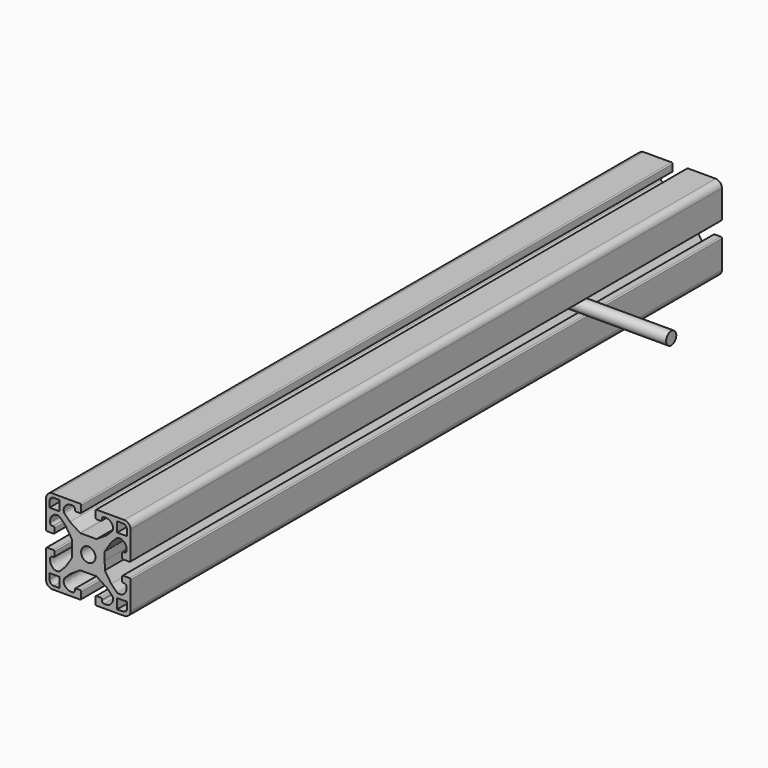
from build123d import *

# Parameters (mm, degrees)
F0_R     = 3.4
F1_DEPTH = 350
F2_R     = 3
F3_DEPTH = 60


with BuildPart() as f1:
    # F0 (on Front) → F1 (new body)
    with BuildSketch(Plane.XZ):
        with BuildLine():
            ThreePointArc((-18.3550221846, 16.3550221846), (-17.7692357469, 17.7692357469), (-16.3550221846, 18.3550221846))
            Line((-16.3550221846, 18.3550221846), (-14.0237337309, 18.3550221846))
            add(Edge.make_bspline(
                [(-14.0237337309, 18.3550221845), (-14.2706563501, 18.8700433502), (-14.531764339, 19.4199819881), (-14.8048075585, 20)],
                knots=[0.5315869177, 0.5315869177, 0.5315869177, 0.5315869177, 0.5531016129, 0.5531016129, 0.5531016129, 0.5531016129], degree=3))
            Line((-14.8048075585, 20), (-17, 20))
            ThreePointArc((-17, 20), (-19.1213203436, 19.1213203436), (-20, 17))
            Line((-20, 17), (-20, 14.8048075585))
            add(Edge.make_bspline(
                [(-18.3550221845, 14.0237337309), (-18.8700433502, 14.2706563501), (-19.4199819881, 14.531764339), (-20, 14.8048075585)],
                knots=[0.5315869177, 0.5315869177, 0.5315869177, 0.5315869177, 0.5531016129, 0.5531016129, 0.5531016129, 0.5531016129], degree=3))
            Line((-18.3550221846, 14.0237337309), (-18.3550221846, 16.3550221846))
        make_face()
        with BuildLine():
            add(Edge.make_bspline(
                [(-14.0237337309, 18.3550221845), (-14.2706563501, 18.8700433502), (-14.531764339, 19.4199819881), (-14.8048075585, 20)],
                knots=[0.5315869177, 0.5315869177, 0.5315869177, 0.5315869177, 0.5531016129, 0.5531016129, 0.5531016129, 0.5531016129], degree=3))
            Line((-14.0237337309, 18.3550221846), (-13.6494976468, 18.3550221846))
            Line((-13.6494976468, 18.3550221846), (-13.6494976468, 17.5788207647))
            add(Edge.make_bspline(
                [(-11.594085993, 14.1061210716), (-11.5738798381, 13.895961995), (-11.5790441073, 13.4753849368), (-12.6022550623, 15.4198368213), (-13.6494976468, 17.5788207647)],
                knots=[0.3845285295, 0.3845285295, 0.3845285295, 0.3845285295, 0.4230558589, 0.5203726283, 0.5203726283, 0.5203726283, 0.5203726283], degree=3))
            add(Edge.make_bspline(
                [(-7.3380557529, 18.077673873), (-7.938915425, 18.114965287), (-9.2671967698, 18.1126101908), (-10.8204009228, 17.1496223508), (-11.7986304949, 15.6154448581), (-11.6169304386, 14.3437203378), (-11.594085993, 14.1061210716)],
                knots=[0.041617921, 0.041617921, 0.041617921, 0.041617921, 0.1226487952, 0.2279423965, 0.3409707382, 0.3845285295, 0.3845285295, 0.3845285295, 0.3845285295], degree=3))
            ThreePointArc((-7.3380557529, 18.077673873), (-6.6713216598, 17.7644503609), (-6.4, 17.0795942618))
            Line((-6.4, 17.0795942618), (-6.4, 16.5))
            ThreePointArc((-6.4, 16.5), (-6.2535533906, 16.1464466094), (-5.9, 16))
            Line((-5.9, 16), (-3.9, 16))
            ThreePointArc((-3.9, 16), (-3.5464466094, 16.1464466094), (-3.4, 16.5))
            Line((-3.4, 16.5), (-3.4, 19.5))
            ThreePointArc((-3.4, 19.5), (-3.5464466094, 19.8535533906), (-3.9, 20))
            Line((-3.9, 20), (-14.8048075585, 20))
        make_face()
        with BuildLine():
            add(Edge.make_bspline(
                [(-11.594085993, 14.1061210716), (-11.5738798381, 13.895961995), (-11.5790441073, 13.4753849368), (-12.6022550623, 15.4198368213), (-13.6494976468, 17.5788207647)],
                knots=[0.3845285295, 0.3845285295, 0.3845285295, 0.3845285295, 0.4230558589, 0.5203726283, 0.5203726283, 0.5203726283, 0.5203726283], degree=3))
            Line((-13.6494976468, 17.5788207647), (-13.6494976468, 13.6494976468))
            Line((-13.6494976468, 13.6494976468), (-17.5788207647, 13.6494976468))
            add(Edge.make_bspline(
                [(-14.1061210716, 11.594085993), (-13.895961995, 11.5738798381), (-13.4753849368, 11.5790441073), (-15.4198368213, 12.6022550623), (-17.5788207647, 13.6494976468)],
                knots=[0.3845285295, 0.3845285295, 0.3845285295, 0.3845285295, 0.4230558589, 0.5203726283, 0.5203726283, 0.5203726283, 0.5203726283], degree=3))
            ThreePointArc((-14.1061210716, 11.594085993), (-13.7753216108, 11.5031614821), (-13.4947198987, 11.3057830914))
            Line((-13.4947198987, 11.3057830914), (-10.8786681667, 8.6897313595))
            Line((-10.8786681667, 8.6897313595), (-7.8307420977, 3.9992546314))
            ThreePointArc((-7.8307420977, 3.9992546314), (-7.7706103093, 3.8688917636), (-7.75, 3.7268159936))
            Line((-7.75, 3.7268159936), (-7.75, -3.7268159936))
            ThreePointArc((-7.75, -3.7268159936), (-7.7706103093, -3.8688917636), (-7.8307420977, -3.9992546314))
            Line((-7.8307420977, -3.9992546314), (-10.8786681667, -8.6897313595))
            Line((-10.8786681667, -8.6897313595), (-13.4947198987, -11.3057830914))
            ThreePointArc((-13.4947198987, -11.3057830914), (-13.7753216108, -11.5031614821), (-14.1061210716, -11.594085993))
            add(Edge.make_bspline(
                [(-14.1061210716, -11.594085993), (-13.895961995, -11.5738798381), (-13.4753849368, -11.5790441073), (-15.4198368213, -12.6022550623), (-17.5788207647, -13.6494976468)],
                knots=[0.3845285295, 0.3845285295, 0.3845285295, 0.3845285295, 0.4230558589, 0.5203726283, 0.5203726283, 0.5203726283, 0.5203726283], degree=3))
            Line((-17.5788207647, -13.6494976468), (-13.6494976468, -13.6494976468))
            Line((-13.6494976468, -13.6494976468), (-13.6494976468, -17.5788207647))
            add(Edge.make_bspline(
                [(-11.594085993, -14.1061210716), (-11.5738798381, -13.895961995), (-11.5790441073, -13.4753849368), (-12.6022550623, -15.4198368213), (-13.6494976468, -17.5788207647)],
                knots=[0.3845285295, 0.3845285295, 0.3845285295, 0.3845285295, 0.4230558589, 0.5203726283, 0.5203726283, 0.5203726283, 0.5203726283], degree=3))
            ThreePointArc((-11.594085993, -14.1061210716), (-11.5031614821, -13.7753216108), (-11.3057830914, -13.4947198987))
            Line((-11.3057830914, -13.4947198987), (-8.6897313595, -10.8786681667))
            Line((-8.6897313595, -10.8786681667), (-3.9992546314, -7.8307420977))
            ThreePointArc((-3.9992546314, -7.8307420977), (-3.8688917636, -7.7706103093), (-3.7268159936, -7.75))
            Line((-3.7268159936, -7.75), (0, -7.75))
            Line((0, -7.75), (3.7268159936, -7.75))
            ThreePointArc((3.7268159936, -7.75), (3.8688917636, -7.7706103093), (3.9992546314, -7.8307420977))
            Line((3.9992546314, -7.8307420977), (8.6897313595, -10.8786681667))
            Line((8.6897313595, -10.8786681667), (11.3057830914, -13.4947198987))
            ThreePointArc((11.3057830914, -13.4947198987), (11.5031614821, -13.7753216108), (11.594085993, -14.1061210716))
            add(Edge.make_bspline(
                [(11.594085993, -14.1061210716), (11.5738798381, -13.895961995), (11.5790441073, -13.4753849368), (12.6022550623, -15.4198368213), (13.6494976468, -17.5788207647)],
                knots=[0.3845285295, 0.3845285295, 0.3845285295, 0.3845285295, 0.4230558589, 0.5203726283, 0.5203726283, 0.5203726283, 0.5203726283], degree=3))
            Line((13.6494976468, -17.5788207647), (13.6494976468, -13.6494976468))
            Line((13.6494976468, -13.6494976468), (17.5788207647, -13.6494976468))
            add(Edge.make_bspline(
                [(14.1061210716, -11.594085993), (13.895961995, -11.5738798381), (13.4753849368, -11.5790441073), (15.4198368213, -12.6022550623), (17.5788207647, -13.6494976468)],
                knots=[0.3845285295, 0.3845285295, 0.3845285295, 0.3845285295, 0.4230558589, 0.5203726283, 0.5203726283, 0.5203726283, 0.5203726283], degree=3))
            ThreePointArc((14.1061210716, -11.594085993), (13.7753216108, -11.5031614821), (13.4947198987, -11.3057830914))
            Line((13.4947198987, -11.3057830914), (10.8786681667, -8.6897313595))
            Line((10.8786681667, -8.6897313595), (7.8307420977, -3.9992546314))
            Line((7.8307420977, -3.9992546314), (7.75, 0))
            Line((7.75, 0), (7.75, 3.7268159936))
            ThreePointArc((7.75, 3.7268159936), (7.7706103093, 3.8688917636), (7.8307420977, 3.9992546314))
            Line((7.8307420977, 3.9992546314), (10.8786681667, 8.6897313595))
            Line((10.8786681667, 8.6897313595), (13.4947198987, 11.3057830914))
            ThreePointArc((13.4947198987, 11.3057830914), (13.7753216108, 11.5031614821), (14.1061210716, 11.594085993))
            add(Edge.make_bspline(
                [(14.1061210716, 11.594085993), (13.895961995, 11.5738798381), (13.4753849368, 11.5790441073), (15.4198368213, 12.6022550623), (17.5788207647, 13.6494976468)],
                knots=[0.3845285295, 0.3845285295, 0.3845285295, 0.3845285295, 0.4230558589, 0.5203726283, 0.5203726283, 0.5203726283, 0.5203726283], degree=3))
            Line((17.5788207647, 13.6494976468), (13.6494976468, 13.6494976468))
            Line((13.6494976468, 13.6494976468), (13.6494976468, 17.5788207647))
            add(Edge.make_bspline(
                [(11.594085993, 14.1061210716), (11.5738798381, 13.895961995), (11.5790441073, 13.4753849368), (12.6022550623, 15.4198368213), (13.6494976468, 17.5788207647)],
                knots=[0.3845285295, 0.3845285295, 0.3845285295, 0.3845285295, 0.4230558589, 0.5203726283, 0.5203726283, 0.5203726283, 0.5203726283], degree=3))
            ThreePointArc((11.594085993, 14.1061210716), (11.5031614821, 13.7753216108), (11.3057830914, 13.4947198987))
            Line((11.3057830914, 13.4947198987), (8.6897313595, 10.8786681667))
            Line((8.6897313595, 10.8786681667), (3.9992546314, 7.8307420977))
            ThreePointArc((3.9992546314, 7.8307420977), (3.8688917636, 7.7706103093), (3.7268159936, 7.75))
            Line((3.7268159936, 7.75), (0, 7.75))
            Line((0, 7.75), (-3.7268159936, 7.75))
            ThreePointArc((-3.7268159936, 7.75), (-3.8688917636, 7.7706103093), (-3.9992546314, 7.8307420977))
            Line((-3.9992546314, 7.8307420977), (-8.6897313595, 10.8786681667))
            Line((-8.6897313595, 10.8786681667), (-11.3057830914, 13.4947198987))
            ThreePointArc((-11.3057830914, 13.4947198987), (-11.5031614821, 13.7753216108), (-11.594085993, 14.1061210716))
        make_face()
        Circle(F0_R, mode=Mode.SUBTRACT)
        with BuildLine():
            Line((-18.3550221846, 13.6494976468), (-18.3550221846, 14.0237337309))
            add(Edge.make_bspline(
                [(-18.3550221845, 14.0237337309), (-18.8700433502, 14.2706563501), (-19.4199819881, 14.531764339), (-20, 14.8048075585)],
                knots=[0.5315869177, 0.5315869177, 0.5315869177, 0.5315869177, 0.5531016129, 0.5531016129, 0.5531016129, 0.5531016129], degree=3))
            Line((-20, 14.8048075585), (-20, 3.9))
            ThreePointArc((-20, 3.9), (-19.8535533906, 3.5464466094), (-19.5, 3.4))
            Line((-19.5, 3.4), (-16.5, 3.4))
            ThreePointArc((-16.5, 3.4), (-16.1464466094, 3.5464466094), (-16, 3.9))
            Line((-16, 3.9), (-16, 5.9))
            ThreePointArc((-16, 5.9), (-16.1464466094, 6.2535533906), (-16.5, 6.4))
            Line((-16.5, 6.4), (-17.0795942618, 6.4))
            ThreePointArc((-17.0795942618, 6.4), (-17.7644503609, 6.6713216598), (-18.077673873, 7.3380557529))
            add(Edge.make_bspline(
                [(-18.077673873, 7.3380557529), (-18.114965287, 7.938915425), (-18.1126101908, 9.2671967698), (-17.1496223508, 10.8204009228), (-15.6154448581, 11.7986304949), (-14.3437203378, 11.6169304386), (-14.1061210716, 11.594085993)],
                knots=[0.041617921, 0.041617921, 0.041617921, 0.041617921, 0.1226487952, 0.2279423965, 0.3409707382, 0.3845285295, 0.3845285295, 0.3845285295, 0.3845285295], degree=3))
            add(Edge.make_bspline(
                [(-14.1061210716, 11.594085993), (-13.895961995, 11.5738798381), (-13.4753849368, 11.5790441073), (-15.4198368213, 12.6022550623), (-17.5788207647, 13.6494976468)],
                knots=[0.3845285295, 0.3845285295, 0.3845285295, 0.3845285295, 0.4230558589, 0.5203726283, 0.5203726283, 0.5203726283, 0.5203726283], degree=3))
            Line((-17.5788207647, 13.6494976468), (-18.3550221846, 13.6494976468))
        make_face()
        with BuildLine():
            add(Edge.make_bspline(
                [(7.3380557529, 18.077673873), (7.938915425, 18.114965287), (9.2671967698, 18.1126101908), (10.8204009228, 17.1496223508), (11.7986304949, 15.6154448581), (11.6169304386, 14.3437203378), (11.594085993, 14.1061210716)],
                knots=[0.041617921, 0.041617921, 0.041617921, 0.041617921, 0.1226487952, 0.2279423965, 0.3409707382, 0.3845285295, 0.3845285295, 0.3845285295, 0.3845285295], degree=3))
            add(Edge.make_bspline(
                [(11.594085993, 14.1061210716), (11.5738798381, 13.895961995), (11.5790441073, 13.4753849368), (12.6022550623, 15.4198368213), (13.6494976468, 17.5788207647)],
                knots=[0.3845285295, 0.3845285295, 0.3845285295, 0.3845285295, 0.4230558589, 0.5203726283, 0.5203726283, 0.5203726283, 0.5203726283], degree=3))
            Line((13.6494976468, 17.5788207647), (13.6494976468, 18.3550221846))
            Line((13.6494976468, 18.3550221846), (14.0237337309, 18.3550221846))
            add(Edge.make_bspline(
                [(14.0237337309, 18.3550221845), (14.2706563501, 18.8700433502), (14.531764339, 19.4199819881), (14.8048075585, 20)],
                knots=[0.5315869177, 0.5315869177, 0.5315869177, 0.5315869177, 0.5531016129, 0.5531016129, 0.5531016129, 0.5531016129], degree=3))
            Line((14.8048075585, 20), (3.9, 20))
            ThreePointArc((3.9, 20), (3.5464466094, 19.8535533906), (3.4, 19.5))
            Line((3.4, 19.5), (3.4, 16.5))
            ThreePointArc((3.4, 16.5), (3.5464466094, 16.1464466094), (3.9, 16))
            Line((3.9, 16), (5.9, 16))
            ThreePointArc((5.9, 16), (6.2535533906, 16.1464466094), (6.4, 16.5))
            Line((6.4, 16.5), (6.4, 17.0795942618))
            ThreePointArc((6.4, 17.0795942618), (6.6713216598, 17.7644503609), (7.3380557529, 18.077673873))
        make_face()
        with BuildLine():
            add(Edge.make_bspline(
                [(-14.1061210716, -11.594085993), (-13.895961995, -11.5738798381), (-13.4753849368, -11.5790441073), (-15.4198368213, -12.6022550623), (-17.5788207647, -13.6494976468)],
                knots=[0.3845285295, 0.3845285295, 0.3845285295, 0.3845285295, 0.4230558589, 0.5203726283, 0.5203726283, 0.5203726283, 0.5203726283], degree=3))
            add(Edge.make_bspline(
                [(-18.077673873, -7.3380557529), (-18.114965287, -7.938915425), (-18.1126101908, -9.2671967698), (-17.1496223508, -10.8204009228), (-15.6154448581, -11.7986304949), (-14.3437203378, -11.6169304386), (-14.1061210716, -11.594085993)],
                knots=[0.041617921, 0.041617921, 0.041617921, 0.041617921, 0.1226487952, 0.2279423965, 0.3409707382, 0.3845285295, 0.3845285295, 0.3845285295, 0.3845285295], degree=3))
            ThreePointArc((-18.077673873, -7.3380557529), (-17.7644503609, -6.6713216598), (-17.0795942618, -6.4))
            Line((-17.0795942618, -6.4), (-16.5, -6.4))
            ThreePointArc((-16.5, -6.4), (-16.1464466094, -6.2535533906), (-16, -5.9))
            Line((-16, -5.9), (-16, -3.9))
            ThreePointArc((-16, -3.9), (-16.1464466094, -3.5464466094), (-16.5, -3.4))
            Line((-16.5, -3.4), (-19.5, -3.4))
            ThreePointArc((-19.5, -3.4), (-19.8535533906, -3.5464466094), (-20, -3.9))
            Line((-20, -3.9), (-20, -14.8048075585))
            add(Edge.make_bspline(
                [(-18.3550221845, -14.0237337309), (-18.8700433502, -14.2706563501), (-19.4199819881, -14.531764339), (-20, -14.8048075585)],
                knots=[0.5315869177, 0.5315869177, 0.5315869177, 0.5315869177, 0.5531016129, 0.5531016129, 0.5531016129, 0.5531016129], degree=3))
            Line((-18.3550221846, -14.0237337309), (-18.3550221846, -13.6494976468))
            Line((-18.3550221846, -13.6494976468), (-17.5788207647, -13.6494976468))
        make_face()
        with BuildLine():
            add(Edge.make_bspline(
                [(14.0237337309, 18.3550221845), (14.2706563501, 18.8700433502), (14.531764339, 19.4199819881), (14.8048075585, 20)],
                knots=[0.5315869177, 0.5315869177, 0.5315869177, 0.5315869177, 0.5531016129, 0.5531016129, 0.5531016129, 0.5531016129], degree=3))
            Line((14.0237337309, 18.3550221846), (16.3550221846, 18.3550221846))
            ThreePointArc((16.3550221846, 18.3550221846), (17.7692357469, 17.7692357469), (18.3550221846, 16.3550221846))
            Line((18.3550221846, 16.3550221846), (18.3550221846, 14.0237337309))
            add(Edge.make_bspline(
                [(18.3550221845, 14.0237337309), (18.8700433502, 14.2706563501), (19.4199819881, 14.531764339), (20, 14.8048075585)],
                knots=[0.5315869177, 0.5315869177, 0.5315869177, 0.5315869177, 0.5531016129, 0.5531016129, 0.5531016129, 0.5531016129], degree=3))
            Line((20, 14.8048075585), (20, 17))
            ThreePointArc((20, 17), (19.1213203436, 19.1213203436), (17, 20))
            Line((17, 20), (14.8048075585, 20))
        make_face()
        with BuildLine():
            Line((-18.3550221846, -16.3550221846), (-18.3550221846, -14.0237337309))
            add(Edge.make_bspline(
                [(-18.3550221845, -14.0237337309), (-18.8700433502, -14.2706563501), (-19.4199819881, -14.531764339), (-20, -14.8048075585)],
                knots=[0.5315869177, 0.5315869177, 0.5315869177, 0.5315869177, 0.5531016129, 0.5531016129, 0.5531016129, 0.5531016129], degree=3))
            Line((-20, -14.8048075585), (-20, -17))
            ThreePointArc((-20, -17), (-19.1213203436, -19.1213203436), (-17, -20))
            Line((-17, -20), (-14.8048075585, -20))
            add(Edge.make_bspline(
                [(-14.0237337309, -18.3550221845), (-14.2706563501, -18.8700433502), (-14.531764339, -19.4199819881), (-14.8048075585, -20)],
                knots=[0.5315869177, 0.5315869177, 0.5315869177, 0.5315869177, 0.5531016129, 0.5531016129, 0.5531016129, 0.5531016129], degree=3))
            Line((-14.0237337309, -18.3550221846), (-16.3550221846, -18.3550221846))
            ThreePointArc((-16.3550221846, -18.3550221846), (-17.7692357469, -17.7692357469), (-18.3550221846, -16.3550221846))
        make_face()
        with BuildLine():
            Line((18.3550221846, 13.6494976468), (17.5788207647, 13.6494976468))
            add(Edge.make_bspline(
                [(14.1061210716, 11.594085993), (13.895961995, 11.5738798381), (13.4753849368, 11.5790441073), (15.4198368213, 12.6022550623), (17.5788207647, 13.6494976468)],
                knots=[0.3845285295, 0.3845285295, 0.3845285295, 0.3845285295, 0.4230558589, 0.5203726283, 0.5203726283, 0.5203726283, 0.5203726283], degree=3))
            add(Edge.make_bspline(
                [(18.077673873, 7.3380557529), (18.114965287, 7.938915425), (18.1126101908, 9.2671967698), (17.1496223508, 10.8204009228), (15.6154448581, 11.7986304949), (14.3437203378, 11.6169304386), (14.1061210716, 11.594085993)],
                knots=[0.041617921, 0.041617921, 0.041617921, 0.041617921, 0.1226487952, 0.2279423965, 0.3409707382, 0.3845285295, 0.3845285295, 0.3845285295, 0.3845285295], degree=3))
            ThreePointArc((18.077673873, 7.3380557529), (17.7644503609, 6.6713216598), (17.0795942618, 6.4))
            Line((17.0795942618, 6.4), (16.5, 6.4))
            ThreePointArc((16.5, 6.4), (16.1464466094, 6.2535533906), (16, 5.9))
            Line((16, 5.9), (16, 3.9))
            ThreePointArc((16, 3.9), (16.1464466094, 3.5464466094), (16.5, 3.4))
            Line((16.5, 3.4), (19.5, 3.4))
            ThreePointArc((19.5, 3.4), (19.8535533906, 3.5464466094), (20, 3.9))
            Line((20, 3.9), (20, 14.8048075585))
            add(Edge.make_bspline(
                [(18.3550221845, 14.0237337309), (18.8700433502, 14.2706563501), (19.4199819881, 14.531764339), (20, 14.8048075585)],
                knots=[0.5315869177, 0.5315869177, 0.5315869177, 0.5315869177, 0.5531016129, 0.5531016129, 0.5531016129, 0.5531016129], degree=3))
            Line((18.3550221846, 14.0237337309), (18.3550221846, 13.6494976468))
        make_face()
        with BuildLine():
            add(Edge.make_bspline(
                [(-11.594085993, -14.1061210716), (-11.5738798381, -13.895961995), (-11.5790441073, -13.4753849368), (-12.6022550623, -15.4198368213), (-13.6494976468, -17.5788207647)],
                knots=[0.3845285295, 0.3845285295, 0.3845285295, 0.3845285295, 0.4230558589, 0.5203726283, 0.5203726283, 0.5203726283, 0.5203726283], degree=3))
            Line((-13.6494976468, -17.5788207647), (-13.6494976468, -18.3550221846))
            Line((-13.6494976468, -18.3550221846), (-14.0237337309, -18.3550221846))
            add(Edge.make_bspline(
                [(-14.0237337309, -18.3550221845), (-14.2706563501, -18.8700433502), (-14.531764339, -19.4199819881), (-14.8048075585, -20)],
                knots=[0.5315869177, 0.5315869177, 0.5315869177, 0.5315869177, 0.5531016129, 0.5531016129, 0.5531016129, 0.5531016129], degree=3))
            Line((-14.8048075585, -20), (-3.9, -20))
            ThreePointArc((-3.9, -20), (-3.5464466094, -19.8535533906), (-3.4, -19.5))
            Line((-3.4, -19.5), (-3.4, -16.5))
            ThreePointArc((-3.4, -16.5), (-3.5464466094, -16.1464466094), (-3.9, -16))
            Line((-3.9, -16), (-5.9, -16))
            ThreePointArc((-5.9, -16), (-6.2535533906, -16.1464466094), (-6.4, -16.5))
            Line((-6.4, -16.5), (-6.4, -17.0795942618))
            ThreePointArc((-6.4, -17.0795942618), (-6.6713216598, -17.7644503609), (-7.3380557529, -18.077673873))
            add(Edge.make_bspline(
                [(-7.3380557529, -18.077673873), (-7.938915425, -18.114965287), (-9.2671967698, -18.1126101908), (-10.8204009228, -17.1496223508), (-11.7986304949, -15.6154448581), (-11.6169304386, -14.3437203378), (-11.594085993, -14.1061210716)],
                knots=[0.041617921, 0.041617921, 0.041617921, 0.041617921, 0.1226487952, 0.2279423965, 0.3409707382, 0.3845285295, 0.3845285295, 0.3845285295, 0.3845285295], degree=3))
        make_face()
        with BuildLine():
            add(Edge.make_bspline(
                [(18.077673873, -7.3380557529), (18.114965287, -7.938915425), (18.1126101908, -9.2671967698), (17.1496223508, -10.8204009228), (15.6154448581, -11.7986304949), (14.3437203378, -11.6169304386), (14.1061210716, -11.594085993)],
                knots=[0.041617921, 0.041617921, 0.041617921, 0.041617921, 0.1226487952, 0.2279423965, 0.3409707382, 0.3845285295, 0.3845285295, 0.3845285295, 0.3845285295], degree=3))
            add(Edge.make_bspline(
                [(14.1061210716, -11.594085993), (13.895961995, -11.5738798381), (13.4753849368, -11.5790441073), (15.4198368213, -12.6022550623), (17.5788207647, -13.6494976468)],
                knots=[0.3845285295, 0.3845285295, 0.3845285295, 0.3845285295, 0.4230558589, 0.5203726283, 0.5203726283, 0.5203726283, 0.5203726283], degree=3))
            Line((17.5788207647, -13.6494976468), (18.3550221846, -13.6494976468))
            Line((18.3550221846, -13.6494976468), (18.3550221846, -14.0237337309))
            add(Edge.make_bspline(
                [(18.3550221845, -14.0237337309), (18.8700433502, -14.2706563501), (19.4199819881, -14.531764339), (20, -14.8048075585)],
                knots=[0.5315869177, 0.5315869177, 0.5315869177, 0.5315869177, 0.5531016129, 0.5531016129, 0.5531016129, 0.5531016129], degree=3))
            Line((20, -14.8048075585), (20, -3.9))
            ThreePointArc((20, -3.9), (19.8535533906, -3.5464466094), (19.5, -3.4))
            Line((19.5, -3.4), (16.5, -3.4))
            ThreePointArc((16.5, -3.4), (16.1464466094, -3.5464466094), (16, -3.9))
            Line((16, -3.9), (16, -5.9))
            ThreePointArc((16, -5.9), (16.1464466094, -6.2535533906), (16.5, -6.4))
            Line((16.5, -6.4), (17.0795942618, -6.4))
            ThreePointArc((17.0795942618, -6.4), (17.7644503609, -6.6713216598), (18.077673873, -7.3380557529))
        make_face()
        with BuildLine():
            add(Edge.make_bspline(
                [(11.594085993, -14.1061210716), (11.5738798381, -13.895961995), (11.5790441073, -13.4753849368), (12.6022550623, -15.4198368213), (13.6494976468, -17.5788207647)],
                knots=[0.3845285295, 0.3845285295, 0.3845285295, 0.3845285295, 0.4230558589, 0.5203726283, 0.5203726283, 0.5203726283, 0.5203726283], degree=3))
            add(Edge.make_bspline(
                [(7.3380557529, -18.077673873), (7.938915425, -18.114965287), (9.2671967698, -18.1126101908), (10.8204009228, -17.1496223508), (11.7986304949, -15.6154448581), (11.6169304386, -14.3437203378), (11.594085993, -14.1061210716)],
                knots=[0.041617921, 0.041617921, 0.041617921, 0.041617921, 0.1226487952, 0.2279423965, 0.3409707382, 0.3845285295, 0.3845285295, 0.3845285295, 0.3845285295], degree=3))
            ThreePointArc((7.3380557529, -18.077673873), (6.6713216598, -17.7644503609), (6.4, -17.0795942618))
            Line((6.4, -17.0795942618), (6.4, -16.5))
            ThreePointArc((6.4, -16.5), (6.2535533906, -16.1464466094), (5.9, -16))
            Line((5.9, -16), (3.9, -16))
            ThreePointArc((3.9, -16), (3.5464466094, -16.1464466094), (3.4, -16.5))
            Line((3.4, -16.5), (3.4, -19.5))
            ThreePointArc((3.4, -19.5), (3.5464466094, -19.8535533906), (3.9, -20))
            Line((3.9, -20), (14.8048075585, -20))
            add(Edge.make_bspline(
                [(14.0237337309, -18.3550221845), (14.2706563501, -18.8700433502), (14.531764339, -19.4199819881), (14.8048075585, -20)],
                knots=[0.5315869177, 0.5315869177, 0.5315869177, 0.5315869177, 0.5531016129, 0.5531016129, 0.5531016129, 0.5531016129], degree=3))
            Line((14.0237337309, -18.3550221846), (13.6494976468, -18.3550221846))
            Line((13.6494976468, -18.3550221846), (13.6494976468, -17.5788207647))
        make_face()
        with BuildLine():
            add(Edge.make_bspline(
                [(18.3550221845, -14.0237337309), (18.8700433502, -14.2706563501), (19.4199819881, -14.531764339), (20, -14.8048075585)],
                knots=[0.5315869177, 0.5315869177, 0.5315869177, 0.5315869177, 0.5531016129, 0.5531016129, 0.5531016129, 0.5531016129], degree=3))
            Line((18.3550221846, -14.0237337309), (18.3550221846, -16.3550221846))
            ThreePointArc((18.3550221846, -16.3550221846), (17.7692357469, -17.7692357469), (16.3550221846, -18.3550221846))
            Line((16.3550221846, -18.3550221846), (14.0237337309, -18.3550221846))
            add(Edge.make_bspline(
                [(14.0237337309, -18.3550221845), (14.2706563501, -18.8700433502), (14.531764339, -19.4199819881), (14.8048075585, -20)],
                knots=[0.5315869177, 0.5315869177, 0.5315869177, 0.5315869177, 0.5531016129, 0.5531016129, 0.5531016129, 0.5531016129], degree=3))
            Line((14.8048075585, -20), (17, -20))
            ThreePointArc((17, -20), (19.1213203436, -19.1213203436), (20, -17))
            Line((20, -17), (20, -14.8048075585))
        make_face()
    extrude(amount=F1_DEPTH)

    # F2 (on Right) → F3 (join)
    with BuildSketch(Plane.YZ):
        with Locations((-80, 0)):
            Circle(F2_R)
    extrude(amount=F3_DEPTH)


solid = f1.part
